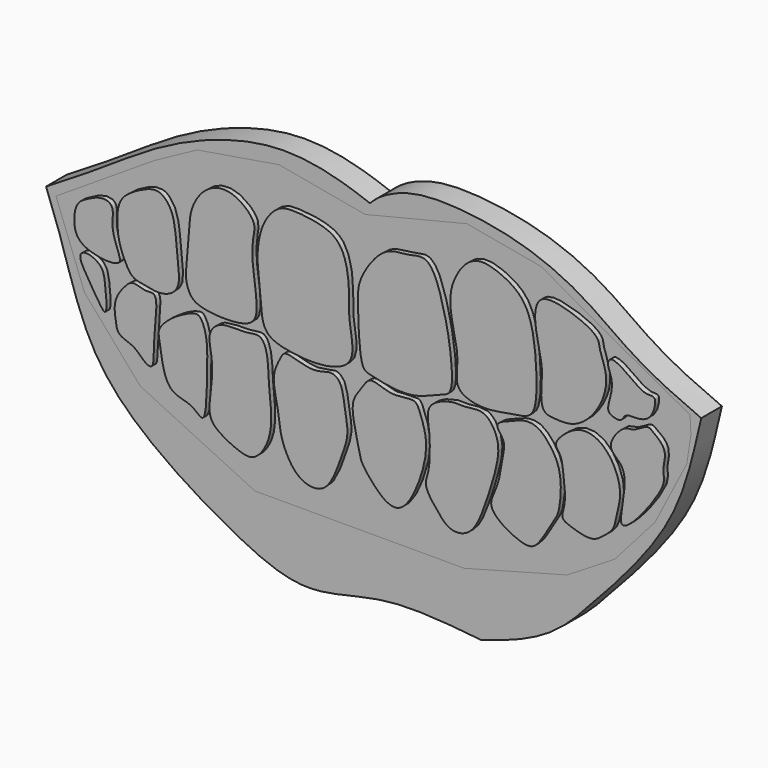
from build123d import *

# Parameters (mm, degrees)
F1_DEPTH = 5
F3_DEPTH = 6
F5_DEPTH = 5


with BuildPart() as f1:
    # F0 (on Front) → F1 (new body)
    with BuildSketch(Plane.XZ):
        with BuildLine():
            add(Edge.make_bspline(
                [(0, 53.1826168299), (11.5920221433, 60.0760877132), (21.3315105261, 68.0243819452), (44.197718028, 76.2956568035), (56.5112424716, 73.0604441818), (62.6554265618, 70.7180127501)],
                knots=[0, 0, 0, 0, 0.3711296272, 0.6948105156, 1, 1, 1, 1], degree=3))
            add(Edge.make_bspline(
                [(0, 53.1826168299), (0.9531224201, 50.6759639912), (3.2183491435, 44.7185582306), (7.8926048175, 27.94217646), (19.3563300179, 15.9271409778), (37.7350566421, 4.7576153385), (50.9985460593, -0.2612043563), (65.5338431133, 5.2522625572), (77.6328001127, 3.9976683477), (84.0732604265, 3.3298286144)],
                knots=[0, 0, 0, 0, 0.1078260071, 0.2562633588, 0.4049781977, 0.5724177914, 0.7054385417, 0.8432004195, 1, 1, 1, 1], degree=3))
            add(Edge.make_bspline(
                [(126.7583326246, 54.956831038), (125.2031178067, 48.4478653643), (122.5974763762, 34.7490205129), (103.4159684392, 14.1917300906), (96.7983826995, 6.9283051416), (84.0732604265, 3.3298286144)],
                knots=[0, 0, 0, 0, 0.3129477921, 0.6585968713, 1, 1, 1, 1], degree=3))
            add(Edge.make_bspline(
                [(126.7583326246, 54.956831038), (122.5783007562, 56.768380437), (114.3425639177, 60.3334502851), (104.0707427451, 68.620671671), (91.9132736526, 73.8681813819), (79.0108606985, 75.7657091263), (69.889826152, 75.4383308974), (64.4772929573, 72.6857344604), (62.6554265618, 70.7180127501)],
                knots=[0, 0, 0, 0, 0.1800748499, 0.3571806098, 0.5355422986, 0.7118174124, 0.8593929672, 1, 1, 1, 1], degree=3))
        make_face()
        with BuildLine():
            add(Edge.make_bspline(
                [(2.9819793999, 52.1809048951), (4.3830942784, 47.9298113056), (7.2946975264, 39.0957762865), (19.773041123, 27.572652256), (30.1316124936, 24.3032467689), (45.5339609419, 16.4493513565), (59.2323865768, 21.1019478784), (67.5450406191, 19.1373347179), (77.6040606742, 20.3220927981), (90.9107116883, 20.5290006915), (107.0973027165, 24.720717209), (123.7517966083, 43.943153815), (123.9046933296, 50.6985535706), (123.9617913961, 53.2213039696)],
                knots=[0, 0, 0, 0, 0.091844252, 0.1908580277, 0.2738015973, 0.3744049699, 0.4660059915, 0.5368540439, 0.6144064509, 0.7040115065, 0.8059796881, 0.9275446551, 1, 1, 1, 1], degree=3))
            add(Edge.make_bspline(
                [(2.9819793999, 52.1809048951), (6.7665438527, 53.8767549325), (14.9559846802, 57.5464146006), (29.5692764688, 68.9354364475), (42.1784077878, 69.7499446437), (59.2914638996, 61.5016088602), (73.4330035148, 69.8375166199), (87.9957183427, 71.3106276065), (102.6692900251, 66.971817544), (119.0124541679, 55.9321137022), (122.69856435, 53.913188158), (123.9617913961, 53.2213039696)],
                knots=[0, 0, 0, 0, 0.1073305941, 0.2322532911, 0.3351774665, 0.4585479705, 0.5743103863, 0.6846022488, 0.802008854, 0.9321485907, 1, 1, 1, 1], degree=3))
        make_face(mode=Mode.SUBTRACT)
    extrude(amount=F1_DEPTH)

    # F2 (on Front) → F3, piece 18 (join)
    with BuildSketch(Plane.XZ):
        with BuildLine():
            add(Edge.make_bspline(
                [(112.4581620097, 32.4393212795), (113.8404944586, 32.3003224585), (121.4478708188, 41.8544010724), (119.7511976548, 44.1184797595), (121.2782372694, 47.9625520086), (118.2115340909, 50.2782650005), (117.0423735974, 51.1221321741), (114.4530579873, 48.9975288856), (112.582121985, 49.6638747357), (108.754585757, 44.8714762168), (112.5247255051, 42.9507961721), (113.1242843604, 38.7980301375), (111.4933432172, 32.5363375036), (112.4581620097, 32.4393212795)],
                knots=[0, 0, 0, 0, 0.1612250224, 0.2391510829, 0.3249789062, 0.4108831938, 0.463116849, 0.5415835506, 0.6058524079, 0.7062458119, 0.7866365527, 0.8874706793, 1, 1, 1, 1], degree=3))
        make_face()
    extrude(amount=F3_DEPTH)


with BuildPart() as f3:
    # F2 (on Front) → F3 (new body)
    with BuildSketch(Plane.XZ):
        with BuildLine():
            add(Edge.make_bspline(
                [(13.5283144191, 54.5306913555), (13.9273906355, 53.7037544286), (13.0552533095, 50.6819175038), (15.3510620154, 46.3614996849), (14.8855791221, 45.2144666611), (12.7382500401, 44.8483770082), (9.0245020548, 45.4882328756), (5.9770774108, 47.4121885031), (6.2366122909, 52.9429743558), (8.6874840741, 54.2998322887), (11.641023108, 55.7685530693), (13.2424342775, 55.1230715476), (13.5283144191, 54.5306913555)],
                knots=[0, 0, 0, 0, 0.1133859596, 0.2396719446, 0.2937067861, 0.3742880227, 0.4880716967, 0.5936281766, 0.7198175378, 0.8148155805, 0.9187754297, 1, 1, 1, 1], degree=3))
        make_face()
    extrude(amount=F3_DEPTH)


with BuildPart() as f3b:
    # F2 (on Front) → F3, piece 2 (new body)
    with BuildSketch(Plane.XZ):
        with BuildLine():
            add(Edge.make_bspline(
                [(15.914382413, 46.4620180428), (16.3600917125, 45.4768431526), (17.3676665398, 43.4587148981), (20.1094371699, 43.3629412409), (22.2744432548, 42.6711877521), (24.988259291, 43.242352078), (26.7753384257, 45.3084166581), (26.3051003534, 49.2955839598), (25.9363562843, 53.3471909257), (25.4097672862, 57.7797243392), (22.7254976965, 60.6382224063), (19.4473687055, 59.5078171431), (15.7779528066, 57.3994425304), (14.4131191191, 54.6301221655), (14.6374973537, 49.5484068912), (15.4500751705, 47.4883009525), (15.914382413, 46.4620180428)],
                knots=[0, 0, 0, 0, 0.0692232328, 0.1308060456, 0.1901564463, 0.2531484356, 0.3140417249, 0.3904561411, 0.4713725588, 0.5539364525, 0.6248773744, 0.6941834924, 0.773923191, 0.8413518524, 0.9278883156, 1, 1, 1, 1], degree=3))
        make_face()
    extrude(amount=F3_DEPTH)


with BuildPart() as f3c:
    # F2 (on Front) → F3, piece 3 (new body)
    with BuildSketch(Plane.XZ):
        with BuildLine():
            add(Edge.make_bspline(
                [(28.6157298833, 44.6893535554), (28.916333948, 44.1833418753), (29.8456946532, 43.1411870333), (34.5797100783, 42.3584454044), (40.7075981978, 42.8066485104), (41.9623712746, 46.303653231), (40.6551085591, 52.8913730276), (40.6499622844, 57.867188428), (41.6470503236, 60.991727745), (37.6774871886, 64.4188132317), (33.9330480551, 64.7833479165), (30.7275606754, 62.8139821268), (28.4898761863, 58.8214293919), (28.4765375649, 53.8999216329), (27.4884430223, 47.3529263213), (28.2464566767, 45.3109571121), (28.6157298833, 44.6893535554)],
                knots=[0, 0, 0, 0, 0.0462908731, 0.1227647118, 0.206535485, 0.2669454189, 0.3577907136, 0.4365597136, 0.495453268, 0.5703964194, 0.6368326367, 0.7020728839, 0.7743834054, 0.8534235592, 0.9431345709, 1, 1, 1, 1], degree=3))
        make_face()
    extrude(amount=F3_DEPTH)


with BuildPart() as f3d:
    # F2 (on Front) → F3, piece 4 (new body)
    with BuildSketch(Plane.XZ):
        with BuildLine():
            add(Edge.make_bspline(
                [(44.520817697, 42.1505123377), (45.4170333596, 41.6317072896), (48.1941700829, 40.9498918311), (54.4648863315, 40.3759569289), (61.1960705476, 42.6916190362), (59.1274324691, 50.2740027304), (59.591457196, 55.3487998558), (58.8119313623, 60.8127781968), (56.265600846, 64.560013379), (48.9133676714, 65.4337844188), (45.6410651911, 65.116423576), (42.3987849268, 61.343881423), (41.3779784851, 55.0730775922), (42.3305845702, 50.1366938409), (42.3997175735, 44.0769824006), (43.766391508, 42.587237706), (44.520817697, 42.1505123377)],
                knots=[0, 0, 0, 0, 0.0608383262, 0.1423586106, 0.2182871824, 0.2998883197, 0.3741288917, 0.4468328505, 0.5118912727, 0.5959456977, 0.6527980402, 0.7199979693, 0.7990415244, 0.8723918379, 0.9487868506, 1, 1, 1, 1], degree=3))
        make_face()
    extrude(amount=F3_DEPTH)


with BuildPart() as f3e:
    # F2 (on Front) → F3, piece 5 (new body)
    with BuildSketch(Plane.XZ):
        with BuildLine():
            add(Edge.make_bspline(
                [(62.0922334492, 43.2368516922), (62.4206105482, 42.4774135409), (63.7446005141, 42.1355398708), (71.1707836501, 40.354608879), (76.6804931701, 43.241114082), (79.556329307, 43.818374356), (79.2595139837, 50.6289226611), (77.8467562909, 58.3905223237), (75.0683520708, 66.4649775316), (70.672823334, 64.6679165815), (66.1085709552, 65.1063540925), (61.0540717623, 57.927824226), (61.133106927, 53.5297911586), (61.3540931488, 44.9439497415), (62.0922334492, 43.2368516922)],
                knots=[0, 0, 0, 0, 0.0491676376, 0.1449169124, 0.2330528009, 0.285986945, 0.3707869858, 0.4771604858, 0.5710091645, 0.6374046906, 0.7112526938, 0.8086206979, 0.8894788495, 1, 1, 1, 1], degree=3))
        make_face()
    extrude(amount=F3_DEPTH)


with BuildPart() as f3f:
    # F2 (on Front) → F3, piece 6 (new body)
    with BuildSketch(Plane.XZ):
        with BuildLine():
            add(Edge.make_bspline(
                [(84.7531706095, 68.3935731649), (83.7147224572, 68.286096193), (81.4990427103, 67.167885558), (78.4448642097, 61.6952858642), (79.4774922409, 55.5078191856), (80.8344081361, 50.1406581722), (79.519652945, 44.8256904343), (85.5812405572, 43.2313960709), (90.4373320611, 44.4916293744), (94.929061895, 44.7745997425), (95.8306757797, 49.054233941), (95.6735779836, 55.5020100293), (94.3723004769, 64.6618816043), (88.6588037449, 67.7965630492), (85.8760935993, 68.5097930864), (84.7531706095, 68.3935731649)],
                knots=[0, 0, 0, 0, 0.0608287224, 0.1426138921, 0.226900743, 0.30753239, 0.3785872724, 0.4539081342, 0.5326253766, 0.5989586041, 0.6626741351, 0.7507548669, 0.8514465139, 0.9342230321, 1, 1, 1, 1], degree=3))
        make_face()
    extrude(amount=F3_DEPTH)


with BuildPart() as f3g:
    # F2 (on Front) → F3, piece 7 (new body)
    with BuildSketch(Plane.XZ):
        with BuildLine():
            add(Edge.make_bspline(
                [(96.7250540853, 52.8628304601), (96.6586811479, 51.2164264355), (96.1307876209, 46.5905185719), (99.435552282, 46.2663747683), (103.7192125767, 46.1417736149), (108.2717554961, 50.9413099936), (109.7835689764, 56.7936525833), (107.7502686696, 60.7730418966), (107.8833671045, 63.0724468533), (102.9075559597, 65.5222934519), (96.9002759881, 66.8133180796), (95.2833991824, 64.0388109826), (95.4542190402, 60.2570203733), (96.5989526793, 55.3909556559), (96.7707250294, 53.9957142725), (96.7250540853, 52.8628304601)],
                knots=[0, 0, 0, 0, 0.0900227327, 0.1496615492, 0.2263539867, 0.3210708718, 0.4132754431, 0.4904099598, 0.5428275516, 0.62971537, 0.7212450457, 0.7802228914, 0.8547340056, 0.9380557293, 1, 1, 1, 1], degree=3))
        make_face()
    extrude(amount=F3_DEPTH)


with BuildPart() as f3h:
    # F2 (on Front) → F3, piece 8 (new body)
    with BuildSketch(Plane.XZ):
        with BuildLine():
            add(Edge.make_bspline(
                [(110.1810261607, 59.9700771272), (111.0512856934, 60.0969822087), (114.2919326745, 57.8324680171), (116.7136710621, 56.0245448626), (118.9619203912, 56.6109295324), (118.4113307194, 53.416504362), (116.909231874, 51.7058777726), (114.5665668717, 51.4669284474), (112.7320373363, 51.6267112807), (112.2423910757, 49.8556471075), (110.081012925, 50.3199073919), (109.2671541873, 51.3152389714), (110.2083786068, 53.9957284915), (110.4389817492, 56.7630269471), (109.2142950519, 58.9122603456), (109.7398576487, 59.9057439899), (110.1810261607, 59.9700771272)],
                knots=[0, 0, 0, 0, 0.1031481172, 0.1917713239, 0.2508374408, 0.3271248152, 0.4011610821, 0.4748893555, 0.5369435189, 0.5941586886, 0.6599136491, 0.7107955293, 0.7903003231, 0.8732827134, 0.9477101949, 1, 1, 1, 1], degree=3))
        make_face()
    extrude(amount=F3_DEPTH)


with BuildPart() as f3i:
    # F2 (on Front) → F3, piece 9 (new body)
    with BuildSketch(Plane.XZ):
        with BuildLine():
            add(Edge.make_bspline(
                [(11.1724650487, 43.887577951), (11.8223338415, 43.252947186), (12.2675515215, 41.5221519165), (12.8150220288, 34.8389662192), (10.7958914754, 37.8211782094), (9.2856177638, 40.162587734), (6.6653733016, 44.4074738812), (8.7437062846, 45.3523382299), (10.5445288397, 44.5007904042), (11.1724650487, 43.887577951)],
                knots=[0, 0, 0, 0, 0.1432714675, 0.3269978142, 0.4354510564, 0.5922458144, 0.7631490086, 0.8615638369, 1, 1, 1, 1], degree=3))
        make_face()
    extrude(amount=F3_DEPTH)


with BuildPart() as f3j:
    # F2 (on Front) → F3, piece 10 (new body)
    with BuildSketch(Plane.XZ):
        with BuildLine():
            add(Edge.make_bspline(
                [(21.1403239518, 29.8340786248), (21.73459449, 30.185525513), (21.3963553106, 34.5757169779), (22.8199931907, 43.0553545962), (20.0081250406, 42.0610042661), (17.5794981514, 43.3566450603), (15.9434465646, 41.7620933952), (13.7484446396, 38.9030684958), (14.2650352643, 35.3129284563), (14.6883822978, 32.9240499241), (17.9275797901, 32.3614736168), (19.4563241655, 30.3540203521), (20.802443289, 29.6342586777), (21.1403239518, 29.8340786248)],
                knots=[0, 0, 0, 0, 0.1140261854, 0.2599797508, 0.3287330076, 0.4116610804, 0.4854523293, 0.584035444, 0.6831093227, 0.7597507551, 0.8489983818, 0.9351688488, 1, 1, 1, 1], degree=3))
        make_face()
    extrude(amount=F3_DEPTH)


with BuildPart() as f3k:
    # F2 (on Front) → F3, piece 11 (new body)
    with BuildSketch(Plane.XZ):
        with BuildLine():
            add(Edge.make_bspline(
                [(30.7342130691, 41.1051101983), (31.1387050854, 40.5545518949), (32.0389068559, 38.1666904026), (31.9711362842, 33.298686527), (31.9208292531, 27.0117361501), (31.2423691573, 23.3448474539), (28.9193969951, 26.3137724509), (23.713105943, 26.1419311107), (22.8828718143, 34.5490834861), (22.2982818998, 36.5871605042), (24.5497568426, 39.044640444), (27.236964173, 40.7237950577), (29.8622856038, 41.846795971), (30.4984741023, 41.4259769654), (30.7342130691, 41.1051101983)],
                knots=[0, 0, 0, 0, 0.0767454916, 0.1789775177, 0.2968512078, 0.3660988908, 0.4371526968, 0.5327702075, 0.6554070452, 0.72119606, 0.7981989375, 0.882425614, 0.955272534, 1, 1, 1, 1], degree=3))
        make_face()
    extrude(amount=F3_DEPTH)


with BuildPart() as f3l:
    # F2 (on Front) → F3, piece 12 (new body)
    with BuildSketch(Plane.XZ):
        with BuildLine():
            add(Edge.make_bspline(
                [(42.2038249671, 41.6820719838), (42.9091117268, 41.312527642), (43.832807227, 38.7841492883), (43.7309889154, 34.1326620926), (45.0935439466, 25.8185565261), (41.5117030872, 20.3027167391), (38.2962686397, 20.7138839417), (33.6396415766, 23.0285802274), (31.7845873358, 25.7682813102), (33.6891477745, 33.8410134492), (31.6557682325, 38.9461143933), (34.5798607268, 41.9806780307), (39.2331076107, 41.244073347), (41.5029798424, 42.0492890721), (42.2038249671, 41.6820719838)],
                knots=[0, 0, 0, 0, 0.0667350249, 0.1532877644, 0.2670856123, 0.3595391985, 0.4249049663, 0.5123358866, 0.5800313039, 0.6903309241, 0.7796329733, 0.8495022219, 0.9336852476, 1, 1, 1, 1], degree=3))
        make_face()
    extrude(amount=F3_DEPTH)


with BuildPart() as f3m:
    # F2 (on Front) → F3, piece 13 (new body)
    with BuildSketch(Plane.XZ):
        with BuildLine():
            add(Edge.make_bspline(
                [(47.2540520132, 40.4698289931), (48.2831401895, 40.5518992477), (52.5203813723, 38.6629880015), (55.9197202796, 40.5917525745), (58.1658340989, 38.8690972362), (58.5278367054, 34.5939874747), (59.4646616072, 30.6269449237), (58.0442771409, 26.812727659), (55.9958397594, 20.7436522214), (53.0599284, 18.9832500096), (48.9725958727, 20.072893996), (46.0866242952, 25.6059777556), (45.8290956512, 30.0536628925), (44.8687302356, 33.9105041754), (44.7291674799, 36.6504196236), (46.2403705895, 39.626193921), (46.7473315296, 40.4294178018), (47.2540520132, 40.4698289931)],
                knots=[0, 0, 0, 0, 0.0789342666, 0.1446868836, 0.1950413066, 0.2656887328, 0.3346683327, 0.4045503906, 0.4909421425, 0.5505660761, 0.6164498168, 0.7003626987, 0.7744672641, 0.8419904867, 0.8993456384, 0.9611329615, 1, 1, 1, 1], degree=3))
        make_face()
    extrude(amount=F3_DEPTH)


with BuildPart() as f3n:
    # F2 (on Front) → F3, piece 14 (new body)
    with BuildSketch(Plane.XZ):
        with BuildLine():
            add(Edge.make_bspline(
                [(62.1043629944, 26.4023970813), (62.7651909502, 25.2936766399), (65.3812656339, 22.0873892134), (68.1752802036, 20.8014708911), (70.5821249628, 21.9836570231), (73.1835782593, 26.9702059848), (74.9823915706, 34.0388367464), (73.1889905124, 38.6893650136), (72.3085559362, 41.1490411624), (67.7079258424, 39.6129386745), (63.4666634839, 42.0995869033), (62.0217275614, 39.4921445972), (59.6728438325, 36.747553427), (60.5077589586, 32.2501057735), (61.471946484, 28.0426280748), (61.7212281906, 27.0452109711), (62.1043629944, 26.4023970813)],
                knots=[0, 0, 0, 0, 0.0851749934, 0.1478318857, 0.2021964965, 0.2886224294, 0.3890433357, 0.4700393343, 0.5210636717, 0.5969306627, 0.6729864304, 0.7286588629, 0.7970020128, 0.8751551515, 0.950617246, 1, 1, 1, 1], degree=3))
        make_face()
    extrude(amount=F3_DEPTH)


with BuildPart() as f3o:
    # F2 (on Front) → F3, piece 15 (new body)
    with BuildSketch(Plane.XZ):
        with BuildLine():
            add(Edge.make_bspline(
                [(75.4973590374, 41.0247668624), (74.7852010102, 40.3328108211), (74.4756414594, 38.5953440848), (75.0997949108, 35.9045704671), (75.0153060241, 32.7875483837), (74.9427739218, 29.2387184471), (73.7527198684, 26.8307275215), (76.2939237819, 23.4302212693), (78.9159131595, 20.3232399422), (83.4612242761, 21.1947238843), (85.6642282923, 27.0552436573), (86.7976150667, 30.4098906603), (88.3432111264, 35.6064111109), (88.4087482522, 39.5672410232), (85.7534549765, 43.553034652), (81.9525490737, 42.4815013268), (79.7942542668, 43.0343808815), (76.44591784, 41.9464176322), (75.4973590374, 41.0247668624)],
                knots=[0, 0, 0, 0, 0.0523677413, 0.1063081709, 0.1648021896, 0.2263317592, 0.2769778995, 0.3420105494, 0.4066970957, 0.4695411419, 0.5487389686, 0.6129870427, 0.6879082134, 0.7538524463, 0.8196640779, 0.8797037042, 0.930248793, 1, 1, 1, 1], degree=3))
        make_face()
    extrude(amount=F3_DEPTH)


with BuildPart() as f3p:
    # F2 (on Front) → F3, piece 16 (new body)
    with BuildSketch(Plane.XZ):
        with BuildLine():
            add(Edge.make_bspline(
                [(88.1232246757, 41.6346043348), (87.9909725882, 41.0386569739), (89.8255788522, 39.4014682767), (89.0233701874, 36.4333537572), (88.5414446266, 31.4827727241), (86.0830454565, 27.623473979), (88.6898478573, 25.1819656751), (90.6523027601, 24.0183072454), (94.4162372701, 22.4277954434), (96.537669989, 24.4271689654), (98.8013469996, 28.7046956316), (100.2060801289, 30.4076516091), (100.7870616907, 37.6166916357), (98.4006958268, 41.5150502333), (95.977578024, 44.0830458422), (93.0839183876, 44.2203903543), (90.9420402066, 43.1349187115), (88.269002748, 42.2915017733), (88.1232246757, 41.6346043348)],
                knots=[0, 0, 0, 0, 0.0528704329, 0.1108443124, 0.1874539511, 0.2555538304, 0.3125071039, 0.3663124161, 0.4304791895, 0.4851555369, 0.5583180828, 0.6101470542, 0.6977778024, 0.7710502257, 0.8323293072, 0.8862666397, 0.9417222825, 1, 1, 1, 1], degree=3))
        make_face()
    extrude(amount=F3_DEPTH)


with BuildPart() as f3q:
    # F2 (on Front) → F3, piece 17 (new body)
    with BuildSketch(Plane.XZ):
        with BuildLine():
            add(Edge.make_bspline(
                [(99.438637495, 41.9765859842), (99.4420131023, 42.6616414341), (101.2332813837, 44.6529766039), (104.3872217461, 46.5167181473), (108.2820994619, 45.5604994176), (111.1817899997, 41.7117813165), (112.2118734389, 37.3854711964), (111.1246716323, 33.653827377), (110.7178979204, 31.0407232668), (108.4799809995, 29.2899885274), (106.4095844146, 27.6711093575), (102.2042792892, 28.9286673231), (100.2584234345, 29.8159127402), (101.4702017744, 32.3894178636), (100.9075592062, 37.2542907016), (100.5309039109, 40.5886233644), (99.4361763765, 41.477119493), (99.438637495, 41.9765859842)],
                knots=[0, 0, 0, 0, 0.0645342327, 0.1363022012, 0.2069578652, 0.2874527422, 0.3657435236, 0.4386159365, 0.4981335477, 0.5590086573, 0.6181327671, 0.6950923827, 0.7436938301, 0.8002339905, 0.8846582439, 0.9529487916, 1, 1, 1, 1], degree=3))
        make_face()
    extrude(amount=F3_DEPTH)


with BuildPart() as f5:
    # F4 (on face) → F5 (new body)
    with BuildSketch(Plane(origin=(0, 0, 0), x_dir=(-1, 0, 0), z_dir=(0, 1, 0))):
        Polygon((-107.3058247566, 64.2345026135), (-124.5828792453, 54.8114255071), (-124.7611120343, 51.4889359474), (-123.9617913961, 46.2597198784), (-117.835201323, 34.363374114), (-110.0207865238, 25.4833530635), (-100.7855534554, 19.8001395911), (-80.8943137527, 14.4721260294), (-40.4014103115, 14.4721260294), (-18.2013567537, 25.1281522214), (-7.4422317557, 37.5264286995), (-1.9165202975, 52.1809048951), (-9.4458032399, 57.0282153785), (-20.9419988096, 64.4281581044), (-29.2248502374, 68.9225643873), (-45.055270195, 71.5606883168), (-61.7300458252, 68.5062929988), (-81.4086571336, 73.3315274119), (-95.7607105374, 70.7180127501), align=None)
    extrude(amount=-F5_DEPTH)


solid = Compound([f1.part, f3.part, f3b.part, f3c.part, f3d.part, f3e.part, f3f.part, f3g.part, f3h.part, f3i.part, f3j.part, f3k.part, f3l.part, f3m.part, f3n.part, f3o.part, f3p.part, f3q.part, f5.part])
